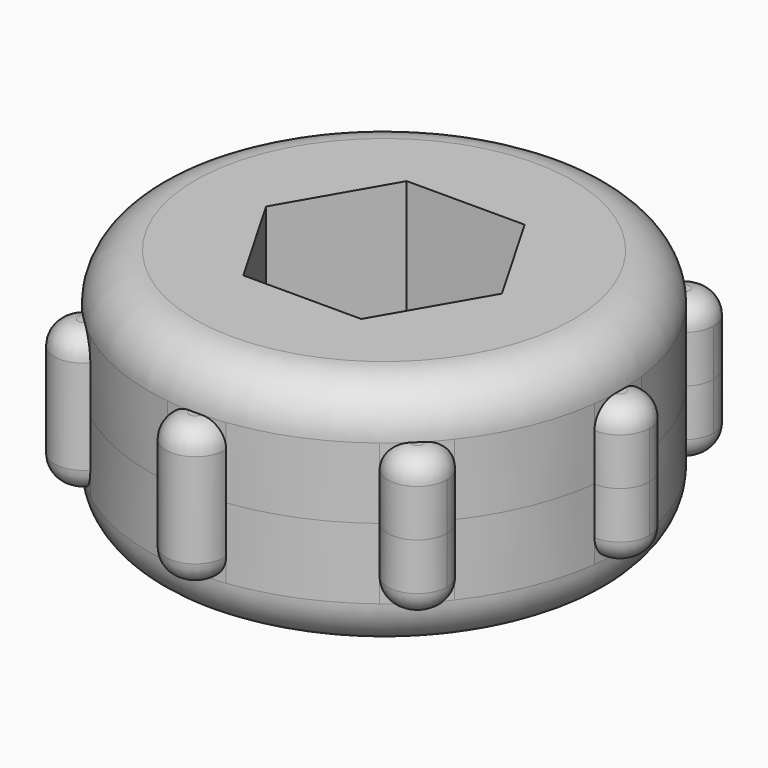
from build123d import *

# Parameters (mm, degrees)
F1_DEPTH     = 12.7
F2_DEPTH     = 7.62
F5_DEPTH     = 19.05
F6_T4_ANGLE  = 359.64
F6_S5_R      = 25.4
F6_T6_DEPTH  = 6
F6_T10_ANGLE = 359.64
F6_S11_R     = 25.4
F6_T12_DEPTH = 6
F6_T16_ANGLE = 359.64
F6_S17_R     = 25.4
F6_T18_DEPTH = 6
F6_T22_ANGLE = 359.64
F6_S23_R     = 25.4
F6_T24_DEPTH = 6
F6_T28_ANGLE = 359.64
F6_S29_R     = 25.4
F6_T30_DEPTH = 6
F6_T34_ANGLE = 359.64
F6_S35_R     = 25.4
F6_T36_DEPTH = 6
F6_T40_ANGLE = 359.64
F6_S41_R     = 25.4
F6_T42_DEPTH = 6
F6_T46_ANGLE = 359.64
F6_S47_R     = 25.4
F6_T48_DEPTH = 6
F6_T52_ANGLE = 359.64
F6_S53_R     = 25.4
F6_T54_DEPTH = 6
F6_T58_ANGLE = 359.64
F6_S59_R     = 25.4
F6_T60_DEPTH = 6
F6_T64_ANGLE = 359.64
F6_S65_R     = 25.4
F6_T66_DEPTH = 6
F6_T70_ANGLE = 359.64
F6_S71_R     = 25.4
F6_T72_DEPTH = 6
F6_T76_ANGLE = 359.64
F6_S77_R     = 25.4
F6_T78_DEPTH = 6
F6_T82_ANGLE = 359.64
F6_S83_R     = 25.4
F6_T84_DEPTH = 6
F6_T88_ANGLE = 359.64
F6_S89_R     = 25.4
F6_T90_DEPTH = 6
F6_T94_ANGLE = 359.64
F6_S95_R     = 25.4
F6_T96_DEPTH = 6


# Not quite as in the source:
# - a fillet or chamfer that OpenCascade refuses, or shapes differently, is made with other operations: its cross-section is extruded or revolved along the edge and cut away or added
# - a feature names something its author has since deleted; it is built from what else it names


with BuildPart() as f1:
    # F0 (on Top) → F1 (new body, symmetric)
    with BuildSketch(Plane.XY):
        with BuildLine():
            ThreePointArc((-20.0608705893, -15.5795208912), (-17.9605122421, -17.9605122421), (-15.5795208912, -20.0608705893))
            ThreePointArc((-15.5795208912, -20.0608705893), (-14.9906408191, -19.0832271349), (-14.7855122421, -17.9605122421))
            ThreePointArc((-14.7855122421, -17.9605122421), (-16.6543753336, -15.0666167056), (-20.0608705893, -15.5795208912))
        make_face()
        with BuildLine():
            ThreePointArc((-3.1687927604, -25.2015625), (0, -25.4), (3.1687927604, -25.2015625))
            ThreePointArc((3.1687927604, -25.2015625), (0, -22.225), (-3.1687927604, -25.2015625))
        make_face()
        with BuildLine():
            ThreePointArc((15.5795208912, -20.0608705893), (17.9605122421, -17.9605122421), (20.0608705893, -15.5795208912))
            ThreePointArc((20.0608705893, -15.5795208912), (15.7154482119, -15.7154482119), (15.5795208912, -20.0608705893))
        make_face()
        with BuildLine():
            ThreePointArc((25.2015625, -3.1687927604), (25.3503420835, -1.5875), (25.4, 0))
            ThreePointArc((25.4, 0), (25.3503420835, 1.5875), (25.2015625, 3.1687927604))
            ThreePointArc((25.2015625, 3.1687927604), (22.225, 0), (25.2015625, -3.1687927604))
        make_face()
        with BuildLine():
            ThreePointArc((15.5795208912, 20.0608705893), (15.7154482119, 15.7154482119), (20.0608705893, 15.5795208912))
            ThreePointArc((20.0608705893, 15.5795208912), (17.9605122421, 17.9605122421), (15.5795208912, 20.0608705893))
        make_face()
        with BuildLine():
            ThreePointArc((-3.1687927604, 25.2015625), (0, 22.225), (3.1687927604, 25.2015625))
            ThreePointArc((3.1687927604, 25.2015625), (0, 25.4), (-3.1687927604, 25.2015625))
        make_face()
        with BuildLine():
            ThreePointArc((-14.7855122421, 17.9605122421), (-14.9906408191, 19.0832271349), (-15.5795208912, 20.0608705893))
            ThreePointArc((-15.5795208912, 20.0608705893), (-17.9605122421, 17.9605122421), (-20.0608705893, 15.5795208912))
            ThreePointArc((-20.0608705893, 15.5795208912), (-16.6543753336, 15.0666167056), (-14.7855122421, 17.9605122421))
        make_face()
        with BuildLine():
            ThreePointArc((-22.225, 0), (-23.0858409667, 2.1737739001), (-25.2015625, 3.1687927604))
            ThreePointArc((-25.2015625, 3.1687927604), (-25.4, 0), (-25.2015625, -3.1687927604))
            ThreePointArc((-25.2015625, -3.1687927604), (-23.0858409667, -2.1737739001), (-22.225, 0))
        make_face()
        with BuildLine():
            ThreePointArc((25.2015625, -3.1687927604), (22.225, 0), (25.2015625, 3.1687927604))
            ThreePointArc((25.2015625, 3.1687927604), (23.4665401258, 9.7201591821), (20.0608705893, 15.5795208912))
            ThreePointArc((20.0608705893, 15.5795208912), (15.7154482119, 15.7154482119), (15.5795208912, 20.0608705893))
            ThreePointArc((15.5795208912, 20.0608705893), (9.7201591821, 23.4665401258), (3.1687927604, 25.2015625))
            ThreePointArc((3.1687927604, 25.2015625), (0, 22.225), (-3.1687927604, 25.2015625))
            ThreePointArc((-3.1687927604, 25.2015625), (-9.7201591821, 23.4665401258), (-15.5795208912, 20.0608705893))
            ThreePointArc((-15.5795208912, 20.0608705893), (-14.9906408191, 19.0832271349), (-14.7855122421, 17.9605122421))
            ThreePointArc((-14.7855122421, 17.9605122421), (-16.6543753336, 15.0666167056), (-20.0608705893, 15.5795208912))
            ThreePointArc((-20.0608705893, 15.5795208912), (-23.4665401258, 9.7201591821), (-25.2015625, 3.1687927604))
            ThreePointArc((-25.2015625, 3.1687927604), (-23.0858409667, 2.1737739001), (-22.225, 0))
            ThreePointArc((-22.225, 0), (-23.0858409667, -2.1737739001), (-25.2015625, -3.1687927604))
            ThreePointArc((-25.2015625, -3.1687927604), (-23.4665401258, -9.7201591821), (-20.0608705893, -15.5795208912))
            ThreePointArc((-20.0608705893, -15.5795208912), (-16.6543753336, -15.0666167056), (-14.7855122421, -17.9605122421))
            ThreePointArc((-14.7855122421, -17.9605122421), (-14.9906408191, -19.0832271349), (-15.5795208912, -20.0608705893))
            ThreePointArc((-15.5795208912, -20.0608705893), (-9.7201591821, -23.4665401258), (-3.1687927604, -25.2015625))
            ThreePointArc((-3.1687927604, -25.2015625), (0, -22.225), (3.1687927604, -25.2015625))
            ThreePointArc((3.1687927604, -25.2015625), (9.7201591821, -23.4665401258), (15.5795208912, -20.0608705893))
            ThreePointArc((15.5795208912, -20.0608705893), (15.7154482119, -15.7154482119), (20.0608705893, -15.5795208912))
            ThreePointArc((20.0608705893, -15.5795208912), (23.4665401258, -9.7201591821), (25.2015625, -3.1687927604))
        make_face()
    extrude(amount=F1_DEPTH, both=True)

    # F0 (on Top) → F2 (join, symmetric)
    with BuildSketch(Plane.XY):
        with BuildLine():
            ThreePointArc((3.175, -25.4), (3.1734478107, -25.3007327204), (3.1687927604, -25.2015625))
            ThreePointArc((3.1687927604, -25.2015625), (0, -25.4), (-3.1687927604, -25.2015625))
            ThreePointArc((-3.1687927604, -25.2015625), (-0.0992672796, -28.5734478107), (3.175, -25.4))
        make_face()
        with BuildLine():
            ThreePointArc((-20.0608705893, -15.5795208912), (-20.2055762724, -20.2055762724), (-15.5795208912, -20.0608705893))
            ThreePointArc((-15.5795208912, -20.0608705893), (-17.9605122421, -17.9605122421), (-20.0608705893, -15.5795208912))
        make_face()
        with BuildLine():
            ThreePointArc((-25.2015625, -3.1687927604), (-25.4, 0), (-25.2015625, 3.1687927604))
            ThreePointArc((-25.2015625, 3.1687927604), (-28.575, 0), (-25.2015625, -3.1687927604))
        make_face()
        with BuildLine():
            ThreePointArc((-20.0608705893, 15.5795208912), (-17.9605122421, 17.9605122421), (-15.5795208912, 20.0608705893))
            ThreePointArc((-15.5795208912, 20.0608705893), (-20.2055762724, 20.2055762724), (-20.0608705893, 15.5795208912))
        make_face()
        with BuildLine():
            ThreePointArc((-3.1687927604, 25.2015625), (0, 25.4), (3.1687927604, 25.2015625))
            ThreePointArc((3.1687927604, 25.2015625), (3.1734478107, 25.3007327204), (3.175, 25.4))
            ThreePointArc((3.175, 25.4), (-0.0992672796, 28.5734478107), (-3.1687927604, 25.2015625))
        make_face()
        with BuildLine():
            ThreePointArc((15.5795208912, 20.0608705893), (17.9605122421, 17.9605122421), (20.0608705893, 15.5795208912))
            ThreePointArc((20.0608705893, 15.5795208912), (20.8544077786, 16.6543753336), (21.1355122421, 17.9605122421))
            ThreePointArc((21.1355122421, 17.9605122421), (19.0832271349, 20.9303836652), (15.5795208912, 20.0608705893))
        make_face()
        with BuildLine():
            ThreePointArc((25.2015625, 3.1687927604), (25.3503420835, 1.5875), (25.4, 0))
            ThreePointArc((25.4, 0), (25.3503420835, -1.5875), (25.2015625, -3.1687927604))
            ThreePointArc((25.2015625, -3.1687927604), (27.5737739001, -2.3141590333), (28.575, 0))
            ThreePointArc((28.575, 0), (27.5737739001, 2.3141590333), (25.2015625, 3.1687927604))
        make_face()
        with BuildLine():
            ThreePointArc((21.1355122421, -17.9605122421), (20.8544077786, -16.6543753336), (20.0608705893, -15.5795208912))
            ThreePointArc((20.0608705893, -15.5795208912), (17.9605122421, -17.9605122421), (15.5795208912, -20.0608705893))
            ThreePointArc((15.5795208912, -20.0608705893), (19.0832271349, -20.9303836652), (21.1355122421, -17.9605122421))
        make_face()
    extrude(amount=F2_DEPTH, both=True)

    # F3: fillet of radius 5.08 on 2 edges, made by hand

    # F3_s1 → F3_t2 (revolve, cut)
    with BuildSketch(Plane(origin=(0, 0, 0), x_dir=(0, 0, 1), z_dir=(-0.7897980547, 0.6133669642, 0))):
        with BuildLine():
            ThreePointArc((-7.62, -25.4), (-11.2121024484, -23.9121024484), (-12.7, -20.32))
            Line((-12.7, -20.32), (-12.7, -25.4))
            Line((-12.7, -25.4), (-7.62, -25.4))
        make_face()
    revolve(axis=Axis((0, 0, -12.7), (0, 0, 1)), mode=Mode.SUBTRACT)

    # F3_s3 → F3_t4 (revolve, cut)
    with BuildSketch(Plane(origin=(0, 0, 0), x_dir=(0, 0, 1), z_dir=(-0.7897980547, 0.6133669642, 0))):
        with BuildLine():
            ThreePointArc((7.62, -25.4), (11.2121024484, -23.9121024484), (12.7, -20.32))
            Line((12.7, -20.32), (12.7, -25.4))
            Line((12.7, -25.4), (7.62, -25.4))
        make_face()
    revolve(axis=Axis((0, 0, 12.7), (0, 0, 1)), mode=Mode.SUBTRACT)

    # F4 (on face) → F5 (cut)
    with BuildSketch(Plane.XY.offset(12.7)):
        Polygon((6.35, 10.9985226281), (-6.35, 10.9985226281), (-12.7, 0), (-6.35, -10.9985226281), (6.35, -10.9985226281), (12.7, 0), align=None)
    extrude(amount=-F5_DEPTH, mode=Mode.SUBTRACT)

    # F6: fillet of radius 2.54 on 16 edges, made by hand


with BuildPart() as f6_tool2:
    # F6_s3 → F6_t4 (revolve)
    with BuildSketch(Plane(origin=(0.0797959284, 0.0002506871, 0), x_dir=(0, 0, 1), z_dir=(-0.9999950652, -0.0031415875, 0))):
        with BuildLine():
            ThreePointArc((7.62, 24.7648746561), (6.8760512242, 22.9688234319), (5.08, 22.2248746561))
            Line((5.08, 22.2248746561), (7.62, 22.2248746561))
            Line((7.62, 22.2248746561), (7.62, 24.7648746561))
        make_face()
    revolve(axis=Axis((0, 25.4, 7.62), (0, 0, 1)), revolution_arc=F6_T4_ANGLE)

    # F6_s5 → F6_t6 (cut, symmetric)
    with BuildSketch(Plane.XY.offset(6.4)):
        Circle(F6_S5_R)
    extrude(amount=F6_T6_DEPTH, both=True, mode=Mode.SUBTRACT)


with BuildPart() as f1_1:
    add(f1.part)

    # F6_t1: cut F6_tool2
    add(f6_tool2.part, mode=Mode.SUBTRACT)


with BuildPart() as f6_tool8:
    # F6_s9 → F6_t10 (revolve)
    with BuildSketch(Plane(origin=(0.0797959284, 0.0002506871, 0), x_dir=(0, 0, 1), z_dir=(-0.9999950652, -0.0031415875, 0))):
        with BuildLine():
            ThreePointArc((-7.62, 24.7648746561), (-6.8760512242, 22.9688234319), (-5.08, 22.2248746561))
            Line((-5.08, 22.2248746561), (-7.62, 22.2248746561))
            Line((-7.62, 22.2248746561), (-7.62, 24.7648746561))
        make_face()
    revolve(axis=Axis((0, 25.4, -7.62), (0, 0, 1)), revolution_arc=F6_T10_ANGLE)

    # F6_s11 → F6_t12 (cut, symmetric)
    with BuildSketch(Plane.XY.offset(-6.4)):
        Circle(F6_S11_R)
    extrude(amount=F6_T12_DEPTH, both=True, mode=Mode.SUBTRACT)


with BuildPart() as f1_2:
    add(f1_1.part)

    # F6_t7: cut F6_tool8
    add(f6_tool8.part, mode=Mode.SUBTRACT)


with BuildPart() as f6_tool14:
    # F6_s15 → F6_t16 (revolve)
    with BuildSketch(Plane(origin=(0.0566015046, -0.0562469795, 0), x_dir=(0, 0, 1), z_dir=(-0.7093247296, 0.7048818539, 0))):
        with BuildLine():
            ThreePointArc((7.62, 24.7648746561), (6.8760512242, 22.9688234319), (5.08, 22.2248746561))
            Line((5.08, 22.2248746561), (7.62, 22.2248746561))
            Line((7.62, 22.2248746561), (7.62, 24.7648746561))
        make_face()
    revolve(axis=Axis((17.9605122421, 17.9605122421, 7.62), (0, 0, 1)), revolution_arc=F6_T16_ANGLE)

    # F6_s17 → F6_t18 (cut, symmetric)
    with BuildSketch(Plane.XY.offset(6.3)):
        Circle(F6_S17_R)
    extrude(amount=F6_T18_DEPTH, both=True, mode=Mode.SUBTRACT)


with BuildPart() as f1_3:
    add(f1_2.part)

    # F6_t13: cut F6_tool14
    add(f6_tool14.part, mode=Mode.SUBTRACT)


with BuildPart() as f6_tool20:
    # F6_s21 → F6_t22 (revolve)
    with BuildSketch(Plane(origin=(0.0566015046, -0.0562469795, 0), x_dir=(0, 0, 1), z_dir=(-0.7093247296, 0.7048818539, 0))):
        with BuildLine():
            ThreePointArc((-7.62, 24.7648746561), (-6.8760512242, 22.9688234319), (-5.08, 22.2248746561))
            Line((-5.08, 22.2248746561), (-7.62, 22.2248746561))
            Line((-7.62, 22.2248746561), (-7.62, 24.7648746561))
        make_face()
    revolve(axis=Axis((17.9605122421, 17.9605122421, -7.62), (0, 0, 1)), revolution_arc=F6_T22_ANGLE)

    # F6_s23 → F6_t24 (cut, symmetric)
    with BuildSketch(Plane.XY.offset(-6.3)):
        Circle(F6_S23_R)
    extrude(amount=F6_T24_DEPTH, both=True, mode=Mode.SUBTRACT)


with BuildPart() as f1_4:
    add(f1_3.part)

    # F6_t19: cut F6_tool20
    add(f6_tool20.part, mode=Mode.SUBTRACT)


with BuildPart() as f6_tool26:
    # F6_s27 → F6_t28 (revolve)
    with BuildSketch(Plane(origin=(0.0562469795, 0.0566015046, 0), x_dir=(0, 0, 1), z_dir=(-0.7048818539, -0.7093247296, 0))):
        with BuildLine():
            ThreePointArc((7.62, 24.7648746561), (6.8760512242, 22.9688234319), (5.08, 22.2248746561))
            Line((5.08, 22.2248746561), (7.62, 22.2248746561))
            Line((7.62, 22.2248746561), (7.62, 24.7648746561))
        make_face()
    revolve(axis=Axis((-17.9605122421, 17.9605122421, 7.62), (0, 0, 1)), revolution_arc=F6_T28_ANGLE)

    # F6_s29 → F6_t30 (cut, symmetric)
    with BuildSketch(Plane.XY.offset(6.3)):
        Circle(F6_S29_R)
    extrude(amount=F6_T30_DEPTH, both=True, mode=Mode.SUBTRACT)


with BuildPart() as f1_5:
    add(f1_4.part)

    # F6_t25: cut F6_tool26
    add(f6_tool26.part, mode=Mode.SUBTRACT)


with BuildPart() as f6_tool32:
    # F6_s33 → F6_t34 (revolve)
    with BuildSketch(Plane(origin=(0.0562469795, 0.0566015046, 0), x_dir=(0, 0, 1), z_dir=(-0.7048818539, -0.7093247296, 0))):
        with BuildLine():
            ThreePointArc((-7.62, 24.7648746561), (-6.8760512242, 22.9688234319), (-5.08, 22.2248746561))
            Line((-5.08, 22.2248746561), (-7.62, 22.2248746561))
            Line((-7.62, 22.2248746561), (-7.62, 24.7648746561))
        make_face()
    revolve(axis=Axis((-17.9605122421, 17.9605122421, -7.62), (0, 0, 1)), revolution_arc=F6_T34_ANGLE)

    # F6_s35 → F6_t36 (cut, symmetric)
    with BuildSketch(Plane.XY.offset(-6.3)):
        Circle(F6_S35_R)
    extrude(amount=F6_T36_DEPTH, both=True, mode=Mode.SUBTRACT)


with BuildPart() as f1_6:
    add(f1_5.part)

    # F6_t31: cut F6_tool32
    add(f6_tool32.part, mode=Mode.SUBTRACT)


with BuildPart() as f6_tool38:
    # F6_s39 → F6_t40 (revolve)
    with BuildSketch(Plane(origin=(0.0002506871, -0.0797959284, 0), x_dir=(0, 0, 1), z_dir=(-0.0031415875, 0.9999950652, 0))):
        with BuildLine():
            ThreePointArc((7.62, 24.7648746561), (6.8760512242, 22.9688234319), (5.08, 22.2248746561))
            Line((5.08, 22.2248746561), (7.62, 22.2248746561))
            Line((7.62, 22.2248746561), (7.62, 24.7648746561))
        make_face()
    revolve(axis=Axis((25.4, 0, 7.62), (0, 0, 1)), revolution_arc=F6_T40_ANGLE)

    # F6_s41 → F6_t42 (cut, symmetric)
    with BuildSketch(Plane.XY.offset(6.4)):
        Circle(F6_S41_R)
    extrude(amount=F6_T42_DEPTH, both=True, mode=Mode.SUBTRACT)


with BuildPart() as f1_7:
    add(f1_6.part)

    # F6_t37: cut F6_tool38
    add(f6_tool38.part, mode=Mode.SUBTRACT)


with BuildPart() as f6_tool44:
    # F6_s45 → F6_t46 (revolve)
    with BuildSketch(Plane(origin=(0.0002506871, -0.0797959284, 0), x_dir=(0, 0, 1), z_dir=(-0.0031415875, 0.9999950652, 0))):
        with BuildLine():
            ThreePointArc((-7.62, 24.7648746561), (-6.8760512242, 22.9688234319), (-5.08, 22.2248746561))
            Line((-5.08, 22.2248746561), (-7.62, 22.2248746561))
            Line((-7.62, 22.2248746561), (-7.62, 24.7648746561))
        make_face()
    revolve(axis=Axis((25.4, 0, -7.62), (0, 0, 1)), revolution_arc=F6_T46_ANGLE)

    # F6_s47 → F6_t48 (cut, symmetric)
    with BuildSketch(Plane.XY.offset(-6.4)):
        Circle(F6_S47_R)
    extrude(amount=F6_T48_DEPTH, both=True, mode=Mode.SUBTRACT)


with BuildPart() as f1_8:
    add(f1_7.part)

    # F6_t43: cut F6_tool44
    add(f6_tool44.part, mode=Mode.SUBTRACT)


with BuildPart() as f6_tool50:
    # F6_s51 → F6_t52 (revolve)
    with BuildSketch(Plane(origin=(-0.0562469795, -0.0566015046, 0), x_dir=(0, 0, 1), z_dir=(0.7048818539, 0.7093247296, 0))):
        with BuildLine():
            ThreePointArc((7.62, 24.7648746561), (6.8760512242, 22.9688234319), (5.08, 22.2248746561))
            Line((5.08, 22.2248746561), (7.62, 22.2248746561))
            Line((7.62, 22.2248746561), (7.62, 24.7648746561))
        make_face()
    revolve(axis=Axis((17.9605122421, -17.9605122421, 7.62), (0, 0, 1)), revolution_arc=F6_T52_ANGLE)

    # F6_s53 → F6_t54 (cut, symmetric)
    with BuildSketch(Plane.XY.offset(6.3)):
        Circle(F6_S53_R)
    extrude(amount=F6_T54_DEPTH, both=True, mode=Mode.SUBTRACT)


with BuildPart() as f1_9:
    add(f1_8.part)

    # F6_t49: cut F6_tool50
    add(f6_tool50.part, mode=Mode.SUBTRACT)


with BuildPart() as f6_tool56:
    # F6_s57 → F6_t58 (revolve)
    with BuildSketch(Plane(origin=(-0.0562469795, -0.0566015046, 0), x_dir=(0, 0, 1), z_dir=(0.7048818539, 0.7093247296, 0))):
        with BuildLine():
            ThreePointArc((-7.62, 24.7648746561), (-6.8760512242, 22.9688234319), (-5.08, 22.2248746561))
            Line((-5.08, 22.2248746561), (-7.62, 22.2248746561))
            Line((-7.62, 22.2248746561), (-7.62, 24.7648746561))
        make_face()
    revolve(axis=Axis((17.9605122421, -17.9605122421, -7.62), (0, 0, 1)), revolution_arc=F6_T58_ANGLE)

    # F6_s59 → F6_t60 (cut, symmetric)
    with BuildSketch(Plane.XY.offset(-6.3)):
        Circle(F6_S59_R)
    extrude(amount=F6_T60_DEPTH, both=True, mode=Mode.SUBTRACT)


with BuildPart() as f1_10:
    add(f1_9.part)

    # F6_t55: cut F6_tool56
    add(f6_tool56.part, mode=Mode.SUBTRACT)


with BuildPart() as f6_tool62:
    # F6_s63 → F6_t64 (revolve)
    with BuildSketch(Plane(origin=(-0.0797959284, -0.0002506871, 0), x_dir=(0, 0, 1), z_dir=(0.9999950652, 0.0031415875, 0))):
        with BuildLine():
            ThreePointArc((5.08, 22.2248746561), (6.8760512242, 22.9688234319), (7.62, 24.7648746561))
            Line((7.62, 24.7648746561), (7.62, 22.2248746561))
            Line((7.62, 22.2248746561), (5.08, 22.2248746561))
        make_face()
    revolve(axis=Axis((0, -25.4, 7.62), (0, 0, 1)), revolution_arc=F6_T64_ANGLE)

    # F6_s65 → F6_t66 (cut, symmetric)
    with BuildSketch(Plane.XY.offset(6.4)):
        Circle(F6_S65_R)
    extrude(amount=F6_T66_DEPTH, both=True, mode=Mode.SUBTRACT)


with BuildPart() as f1_11:
    add(f1_10.part)

    # F6_t61: cut F6_tool62
    add(f6_tool62.part, mode=Mode.SUBTRACT)


with BuildPart() as f6_tool68:
    # F6_s69 → F6_t70 (revolve)
    with BuildSketch(Plane(origin=(-0.0797959284, -0.0002506871, 0), x_dir=(0, 0, 1), z_dir=(0.9999950652, 0.0031415875, 0))):
        with BuildLine():
            ThreePointArc((-5.08, 22.2248746561), (-6.8760512242, 22.9688234319), (-7.62, 24.7648746561))
            Line((-7.62, 24.7648746561), (-7.62, 22.2248746561))
            Line((-7.62, 22.2248746561), (-5.08, 22.2248746561))
        make_face()
    revolve(axis=Axis((0, -25.4, -7.62), (0, 0, 1)), revolution_arc=F6_T70_ANGLE)

    # F6_s71 → F6_t72 (cut, symmetric)
    with BuildSketch(Plane.XY.offset(-6.4)):
        Circle(F6_S71_R)
    extrude(amount=F6_T72_DEPTH, both=True, mode=Mode.SUBTRACT)


with BuildPart() as f1_12:
    add(f1_11.part)

    # F6_t67: cut F6_tool68
    add(f6_tool68.part, mode=Mode.SUBTRACT)


with BuildPart() as f6_tool74:
    # F6_s75 → F6_t76 (revolve)
    with BuildSketch(Plane(origin=(-0.0566015046, 0.0562469795, 0), x_dir=(0, 0, 1), z_dir=(0.7093247296, -0.7048818539, 0))):
        with BuildLine():
            ThreePointArc((5.08, 22.2248746561), (6.8760512242, 22.9688234319), (7.62, 24.7648746561))
            Line((7.62, 24.7648746561), (7.62, 22.2248746561))
            Line((7.62, 22.2248746561), (5.08, 22.2248746561))
        make_face()
    revolve(axis=Axis((-17.9605122421, -17.9605122421, 7.62), (0, 0, 1)), revolution_arc=F6_T76_ANGLE)

    # F6_s77 → F6_t78 (cut, symmetric)
    with BuildSketch(Plane.XY.offset(6.4)):
        Circle(F6_S77_R)
    extrude(amount=F6_T78_DEPTH, both=True, mode=Mode.SUBTRACT)


with BuildPart() as f1_13:
    add(f1_12.part)

    # F6_t73: cut F6_tool74
    add(f6_tool74.part, mode=Mode.SUBTRACT)


with BuildPart() as f6_tool80:
    # F6_s81 → F6_t82 (revolve)
    with BuildSketch(Plane(origin=(-0.0566015046, 0.0562469795, 0), x_dir=(0, 0, 1), z_dir=(0.7093247296, -0.7048818539, 0))):
        with BuildLine():
            ThreePointArc((-5.08, 22.2248746561), (-6.8760512242, 22.9688234319), (-7.62, 24.7648746561))
            Line((-7.62, 24.7648746561), (-7.62, 22.2248746561))
            Line((-7.62, 22.2248746561), (-5.08, 22.2248746561))
        make_face()
    revolve(axis=Axis((-17.9605122421, -17.9605122421, -7.62), (0, 0, 1)), revolution_arc=F6_T82_ANGLE)

    # F6_s83 → F6_t84 (cut, symmetric)
    with BuildSketch(Plane.XY.offset(-6.4)):
        Circle(F6_S83_R)
    extrude(amount=F6_T84_DEPTH, both=True, mode=Mode.SUBTRACT)


with BuildPart() as f1_14:
    add(f1_13.part)

    # F6_t79: cut F6_tool80
    add(f6_tool80.part, mode=Mode.SUBTRACT)


with BuildPart() as f6_tool86:
    # F6_s87 → F6_t88 (revolve)
    with BuildSketch(Plane(origin=(-0.0002506871, 0.0797959284, 0), x_dir=(0, 0, 1), z_dir=(0.0031415875, -0.9999950652, 0))):
        with BuildLine():
            ThreePointArc((7.62, 24.7648746561), (6.8760512242, 22.9688234319), (5.08, 22.2248746561))
            Line((5.08, 22.2248746561), (7.62, 22.2248746561))
            Line((7.62, 22.2248746561), (7.62, 24.7648746561))
        make_face()
    revolve(axis=Axis((-25.4, 0, 7.62), (0, 0, 1)), revolution_arc=F6_T88_ANGLE)

    # F6_s89 → F6_t90 (cut, symmetric)
    with BuildSketch(Plane.XY.offset(6.4)):
        Circle(F6_S89_R)
    extrude(amount=F6_T90_DEPTH, both=True, mode=Mode.SUBTRACT)


with BuildPart() as f1_15:
    add(f1_14.part)

    # F6_t85: cut F6_tool86
    add(f6_tool86.part, mode=Mode.SUBTRACT)


with BuildPart() as f6_tool92:
    # F6_s93 → F6_t94 (revolve)
    with BuildSketch(Plane(origin=(-0.0002506871, 0.0797959284, 0), x_dir=(0, 0, 1), z_dir=(0.0031415875, -0.9999950652, 0))):
        with BuildLine():
            ThreePointArc((-7.62, 24.7648746561), (-6.8760512242, 22.9688234319), (-5.08, 22.2248746561))
            Line((-5.08, 22.2248746561), (-7.62, 22.2248746561))
            Line((-7.62, 22.2248746561), (-7.62, 24.7648746561))
        make_face()
    revolve(axis=Axis((-25.4, 0, -7.62), (0, 0, 1)), revolution_arc=F6_T94_ANGLE)

    # F6_s95 → F6_t96 (cut, symmetric)
    with BuildSketch(Plane.XY.offset(-6.4)):
        Circle(F6_S95_R)
    extrude(amount=F6_T96_DEPTH, both=True, mode=Mode.SUBTRACT)


with BuildPart() as f1_16:
    add(f1_15.part)

    # F6_t91: cut F6_tool92
    add(f6_tool92.part, mode=Mode.SUBTRACT)


solid = f1_16.part
